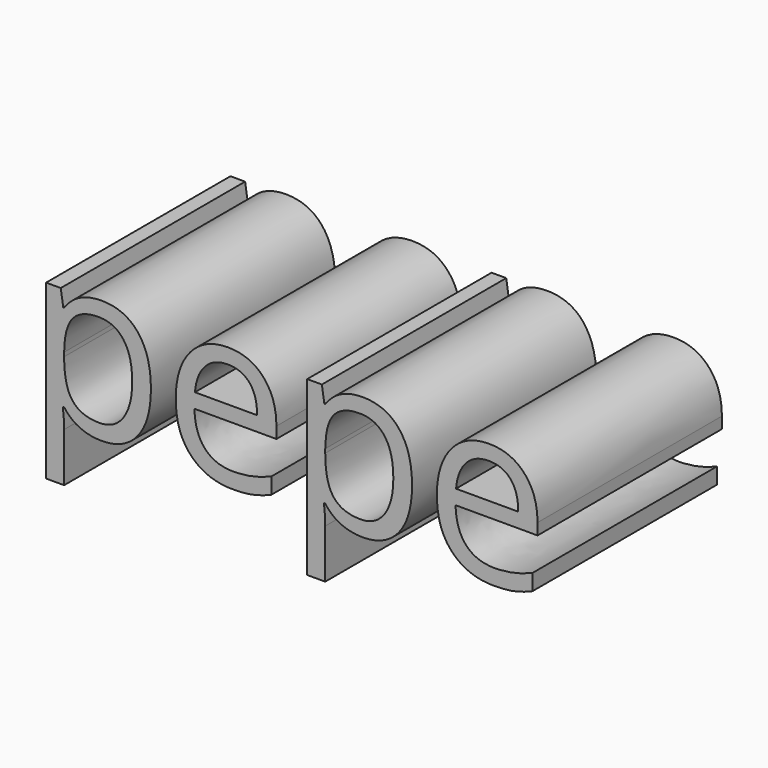
from build123d import *

# Parameters (mm, degrees)
F0_TEXT_SIZE = 38.6078759568
F1_DEPTH     = 40


# Not quite as in the source:
# - Text() gives the source's letters only with a copy of the font that has no kerning and outlines rounded to 1/6400 em; it was checked with that copy


with BuildPart() as f1:
    # F0 (on Front) → F1 (new body)
    with BuildSketch(Plane.XZ):
        with Locations((-91.1266522192, 9.7367115054)):
            Text('pepe', F0_TEXT_SIZE, font='Open Sans', text_align=(TextAlign.LEFT, TextAlign.BOTTOM))
    extrude(amount=F1_DEPTH)


solid = f1.part
